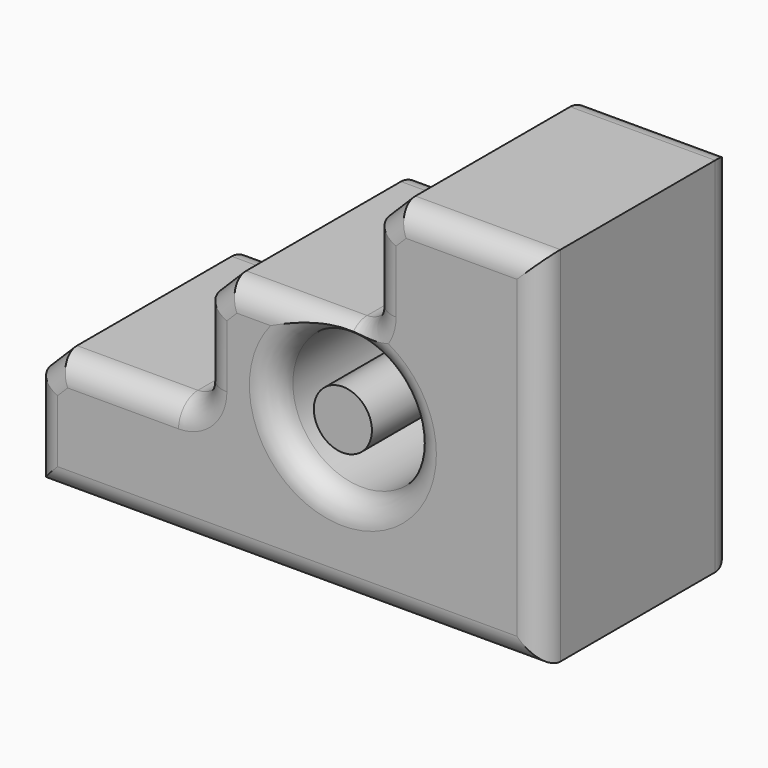
from build123d import *

# Parameters (mm, degrees)
F1_DEPTH     = 25
F2_R         = 14.3434394771
F2_R_2       = 6.0096705541
F3_DEPTH     = 50
F4_SIZE      = 5
F5_T1_DEPTH  = 55
F5_T3_DEPTH  = 32.0710678119
F5_T5_DEPTH  = 27.5
F5_T7_DEPTH  = 32.0710678119
F5_T9_DEPTH  = 27.5
F5_T11_DEPTH = 37.5
F5_T13_DEPTH = 37.5
F5_T15_DEPTH = 32.0710678119
F5_T17_DEPTH = 45
F5_T19_DEPTH = 130
F5_T21_DEPTH = 100
F5_T24_ANGLE = 90
F5_T26_ANGLE = 90
F5_T30_ANGLE = 90
F5_T32_ANGLE = 90


# Not quite as in the source:
# - a fillet or chamfer that OpenCascade refuses, or shapes differently, is made with other operations: its cross-section is extruded or revolved along the edge and cut away or added


with BuildPart() as f1:
    # F0 (on Front) → F1 (new body, symmetric)
    with BuildSketch(Plane.XZ):
        with BuildLine():
            Line((-45.1239673958, 25), (-45.1239673958, 0))
            Line((-45.1239673958, 0), (59.8760326042, 0))
            Line((59.8760326042, 0), (59.8760326042, 75))
            Line((59.8760326042, 75), (24.8760326042, 75))
            Line((24.8760326042, 75), (24.8760326042, 55))
            ThreePointArc((24.8760326042, 55), (23.4115665102, 51.4644660941), (19.8760326042, 50))
            Line((19.8760326042, 50), (-10.1239673958, 50))
            Line((-10.1239673958, 50), (-10.1239673958, 30))
            ThreePointArc((-10.1239673958, 30), (-11.5884334898, 26.4644660941), (-15.1239673958, 25))
            Line((-15.1239673958, 25), (-45.1239673958, 25))
        make_face()
    extrude(amount=F1_DEPTH, both=True)

    # F2 (on face) → F3 (cut, through all)
    with BuildSketch(Plane.XZ.offset(25)):
        with Locations((18.8663620502, 32.7215865254)):
            Circle(F2_R)
        with Locations((18.8663620502, 32.7215865254)):
            Circle(F2_R_2, mode=Mode.SUBTRACT)
    extrude(amount=-F3_DEPTH, mode=Mode.SUBTRACT)

    # F4
    f4_edges = [f1.edges().sort_by_distance(p)[0] for p in [
        (-45.123967, 0, 25),
        (-10.123967, 0, 50),
        (24.876033, 0, 75),
    ]]
    chamfer(f4_edges, length=F4_SIZE)

    # F5: fillet of radius 5 on 28 edges, made by hand

    # F5_s2 → F5_t1 (cut)
    with BuildSketch(Plane.YZ.offset(17.3760326042)):
        with BuildLine():
            ThreePointArc((-20, 75), (-23.5355339059, 73.5355339059), (-25, 70))
            Line((-25, 70), (-25, 75))
            Line((-25, 75), (-20, 75))
        make_face()
        with BuildLine():
            ThreePointArc((25, 70), (23.5355339059, 73.5355339059), (20, 75))
            Line((20, 75), (25, 75))
            Line((25, 75), (25, 70))
        make_face()
    extrude(amount=F5_T1_DEPTH, mode=Mode.SUBTRACT)

    # F5_s4 → F5_t3 (cut)
    with BuildSketch(Plane(origin=(38.5991815373, 0, 38.5991815373), x_dir=(0, 1, 0), z_dir=(0.7071067812, 0, 0.7071067812))):
        with BuildLine():
            ThreePointArc((-20, 31.9074633396), (-23.5355339059, 30.4429972455), (-25, 26.9074633396))
            Line((-25, 26.9074633396), (-25, 31.9074633396))
            Line((-25, 31.9074633396), (-20, 31.9074633396))
        make_face()
        with BuildLine():
            ThreePointArc((25, 26.9074633396), (23.5355339059, 30.4429972455), (20, 31.9074633396))
            Line((20, 31.9074633396), (25, 31.9074633396))
            Line((25, 31.9074633396), (25, 26.9074633396))
        make_face()
    extrude(amount=F5_T3_DEPTH, mode=Mode.SUBTRACT)

    # F5_s6 → F5_t5 (cut)
    with BuildSketch(Plane.XY.offset(55)):
        with BuildLine():
            ThreePointArc((24.8760326042, -20), (26.3404986983, -23.5355339059), (29.8760326042, -25))
            Line((29.8760326042, -25), (24.8760326042, -25))
            Line((24.8760326042, -25), (24.8760326042, -20))
        make_face()
        with BuildLine():
            ThreePointArc((29.8760326042, 25), (26.3404986983, 23.5355339059), (24.8760326042, 20))
            Line((24.8760326042, 20), (24.8760326042, 25))
            Line((24.8760326042, 25), (29.8760326042, 25))
        make_face()
    extrude(amount=F5_T5_DEPTH, mode=Mode.SUBTRACT)

    # F5_s8 → F5_t7 (cut)
    with BuildSketch(Plane(origin=(8.5991815373, 0, 8.5991815373), x_dir=(0, 1, 0), z_dir=(0.7071067812, 0, 0.7071067812))):
        with BuildLine():
            ThreePointArc((-20, 38.9785311515), (-23.5355339059, 37.5140650574), (-25, 33.9785311515))
            Line((-25, 33.9785311515), (-25, 38.9785311515))
            Line((-25, 38.9785311515), (-20, 38.9785311515))
        make_face()
        with BuildLine():
            ThreePointArc((25, 33.9785311515), (23.5355339059, 37.5140650574), (20, 38.9785311515))
            Line((20, 38.9785311515), (25, 38.9785311515))
            Line((25, 38.9785311515), (25, 33.9785311515))
        make_face()
    extrude(amount=F5_T7_DEPTH, mode=Mode.SUBTRACT)

    # F5_s10 → F5_t9 (cut)
    with BuildSketch(Plane.XY.offset(30)):
        with BuildLine():
            ThreePointArc((-10.1239673958, -20), (-8.6595013017, -23.5355339059), (-5.1239673958, -25))
            Line((-5.1239673958, -25), (-10.1239673958, -25))
            Line((-10.1239673958, -25), (-10.1239673958, -20))
        make_face()
        with BuildLine():
            ThreePointArc((-5.1239673958, 25), (-8.6595013017, 23.5355339059), (-10.1239673958, 20))
            Line((-10.1239673958, 20), (-10.1239673958, 25))
            Line((-10.1239673958, 25), (-5.1239673958, 25))
        make_face()
    extrude(amount=F5_T9_DEPTH, mode=Mode.SUBTRACT)

    # F5_s12 → F5_t11 (cut)
    with BuildSketch(Plane.YZ.offset(-17.6239673958)):
        with BuildLine():
            ThreePointArc((-20, 50), (-23.5355339059, 48.5355339059), (-25, 45))
            Line((-25, 45), (-25, 50))
            Line((-25, 50), (-20, 50))
        make_face()
        with BuildLine():
            ThreePointArc((25, 45), (23.5355339059, 48.5355339059), (20, 50))
            Line((20, 50), (25, 50))
            Line((25, 50), (25, 45))
        make_face()
    extrude(amount=F5_T11_DEPTH, mode=Mode.SUBTRACT)

    # F5_s14 → F5_t13 (cut)
    with BuildSketch(Plane.YZ.offset(-52.6239673958)):
        with BuildLine():
            ThreePointArc((-20, 25), (-23.5355339059, 23.5355339059), (-25, 20))
            Line((-25, 20), (-25, 25))
            Line((-25, 25), (-20, 25))
        make_face()
        with BuildLine():
            ThreePointArc((25, 20), (23.5355339059, 23.5355339059), (20, 25))
            Line((20, 25), (25, 25))
            Line((25, 25), (25, 20))
        make_face()
    extrude(amount=F5_T13_DEPTH, mode=Mode.SUBTRACT)

    # F5_s16 → F5_t15 (cut)
    with BuildSketch(Plane(origin=(1.2768510669, 0, 1.2768510669), x_dir=(0, 1, 0), z_dir=(-0.7071067812, 0, -0.7071067812))):
        with BuildLine():
            ThreePointArc((-20, -46.0495989633), (-23.5355339059, -44.5851328693), (-25, -41.0495989633))
            Line((-25, -41.0495989633), (-25, -46.0495989633))
            Line((-25, -46.0495989633), (-20, -46.0495989633))
        make_face()
        with BuildLine():
            ThreePointArc((25, -41.0495989633), (23.5355339059, -44.5851328693), (20, -46.0495989633))
            Line((20, -46.0495989633), (25, -46.0495989633))
            Line((25, -46.0495989633), (25, -41.0495989633))
        make_face()
    extrude(amount=F5_T15_DEPTH, mode=Mode.SUBTRACT)

    # F5_s18 → F5_t17 (cut)
    with BuildSketch(Plane.XY.offset(-12.5)):
        with BuildLine():
            ThreePointArc((-45.1239673958, -20), (-43.6595013017, -23.5355339059), (-40.1239673958, -25))
            Line((-40.1239673958, -25), (-45.1239673958, -25))
            Line((-45.1239673958, -25), (-45.1239673958, -20))
        make_face()
        with BuildLine():
            ThreePointArc((-40.1239673958, 25), (-43.6595013017, 23.5355339059), (-45.1239673958, 20))
            Line((-45.1239673958, 20), (-45.1239673958, 25))
            Line((-45.1239673958, 25), (-40.1239673958, 25))
        make_face()
    extrude(amount=F5_T17_DEPTH, mode=Mode.SUBTRACT)

    # F5_s20 → F5_t19 (cut)
    with BuildSketch(Plane.YZ.offset(-57.6239673958)):
        with BuildLine():
            ThreePointArc((-20, 0), (-23.5355339059, 1.4644660941), (-25, 5))
            Line((-25, 5), (-25, 0))
            Line((-25, 0), (-20, 0))
        make_face()
        with BuildLine():
            ThreePointArc((25, 5), (23.5355339059, 1.4644660941), (20, 0))
            Line((20, 0), (25, 0))
            Line((25, 0), (25, 5))
        make_face()
    extrude(amount=F5_T19_DEPTH, mode=Mode.SUBTRACT)

    # F5_s22 → F5_t21 (cut)
    with BuildSketch(Plane.XY.offset(-12.5)):
        with BuildLine():
            ThreePointArc((59.8760326042, -20), (58.4115665102, -23.5355339059), (54.8760326042, -25))
            Line((54.8760326042, -25), (59.8760326042, -25))
            Line((59.8760326042, -25), (59.8760326042, -20))
        make_face()
        with BuildLine():
            ThreePointArc((54.8760326042, 25), (58.4115665102, 23.5355339059), (59.8760326042, 20))
            Line((59.8760326042, 20), (59.8760326042, 25))
            Line((59.8760326042, 25), (54.8760326042, 25))
        make_face()
    extrude(amount=F5_T21_DEPTH, mode=Mode.SUBTRACT)

    # F5_s23 → F5_t24 (revolve, cut)
    with BuildSketch(Plane.XY.offset(55)):
        with BuildLine():
            ThreePointArc((24.8760326042, -20), (26.3404986983, -23.5355339059), (29.8760326042, -25))
            Line((29.8760326042, -25), (24.8760326042, -25))
            Line((24.8760326042, -25), (24.8760326042, -20))
        make_face()
    revolve(axis=Axis((19.8760326042, -25, 55), (0, 1, 0)), revolution_arc=F5_T24_ANGLE, mode=Mode.SUBTRACT)

    # F5_s25 → F5_t26 (revolve, cut)
    with BuildSketch(Plane.XY.offset(30)):
        with BuildLine():
            ThreePointArc((-10.1239673958, -20), (-8.6595013017, -23.5355339059), (-5.1239673958, -25))
            Line((-5.1239673958, -25), (-10.1239673958, -25))
            Line((-10.1239673958, -25), (-10.1239673958, -20))
        make_face()
    revolve(axis=Axis((-15.1239673958, -25, 30), (0, 1, 0)), revolution_arc=F5_T26_ANGLE, mode=Mode.SUBTRACT)

    # F5_s27 → F5_t28 (revolve, cut)
    with BuildSketch(Plane.XY.offset(32.7215865254)):
        with BuildLine():
            ThreePointArc((33.2098015273, -20), (34.6742676213, -23.5355339059), (38.2098015273, -25))
            Line((38.2098015273, -25), (33.2098015273, -25))
            Line((33.2098015273, -25), (33.2098015273, -20))
        make_face()
    revolve(axis=Axis((18.8663620502, -25, 32.7215865254), (0, -1, 0)), mode=Mode.SUBTRACT)

    # F5_s29 → F5_t30 (revolve, cut)
    with BuildSketch(Plane.XY.offset(30)):
        with BuildLine():
            ThreePointArc((-5.1239673958, 25), (-8.6595013017, 23.5355339059), (-10.1239673958, 20))
            Line((-10.1239673958, 20), (-10.1239673958, 25))
            Line((-10.1239673958, 25), (-5.1239673958, 25))
        make_face()
    revolve(axis=Axis((-15.1239673958, 25, 30), (0, 1, 0)), revolution_arc=F5_T30_ANGLE, mode=Mode.SUBTRACT)

    # F5_s31 → F5_t32 (revolve, cut)
    with BuildSketch(Plane.XY.offset(55)):
        with BuildLine():
            ThreePointArc((29.8760326042, 25), (26.3404986983, 23.5355339059), (24.8760326042, 20))
            Line((24.8760326042, 20), (24.8760326042, 25))
            Line((24.8760326042, 25), (29.8760326042, 25))
        make_face()
    revolve(axis=Axis((19.8760326042, 25, 55), (0, 1, 0)), revolution_arc=F5_T32_ANGLE, mode=Mode.SUBTRACT)

    # F5_s33 → F5_t34 (revolve, cut)
    with BuildSketch(Plane.XY.offset(32.7215865254)):
        with BuildLine():
            ThreePointArc((38.2098015273, 25), (34.6742676213, 23.5355339059), (33.2098015273, 20))
            Line((33.2098015273, 20), (33.2098015273, 25))
            Line((33.2098015273, 25), (38.2098015273, 25))
        make_face()
    revolve(axis=Axis((18.8663620502, 25, 32.7215865254), (0, -1, 0)), mode=Mode.SUBTRACT)


solid = f1.part
